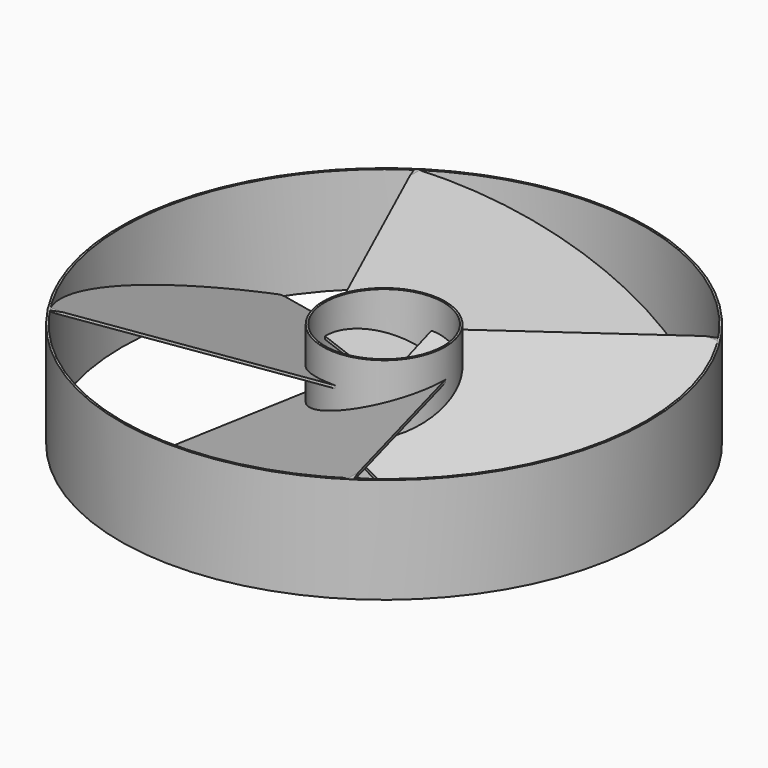
from build123d import *

# Parameters (mm, degrees)
F0_R      = 23.25
F0_R_2    = 22.5
F1_DEPTH  = 140
F3_R      = 100.25
F3_R_2    = 99.5
F4_DEPTH  = 40
F6_REACH  = 217.271158112
F8_DEPTH  = 50
F10_DEPTH = 150
F11_COUNT = 4
F14_ANGLE = 180
F15_R     = 43.2298787394
F16_DEPTH = 100


with BuildPart() as f1:
    # F0 (on Top) → F1 (new body)
    with BuildSketch(Plane.XY):
        Circle(F0_R)
        Circle(F0_R_2, mode=Mode.SUBTRACT)
    extrude(amount=F1_DEPTH)


with BuildPart() as f4:
    # F3 (on offset) → F4 (new body)
    with BuildSketch(Plane.XY.offset(140)):
        Circle(F3_R)
        Circle(F3_R_2, mode=Mode.SUBTRACT)
    extrude(amount=-F4_DEPTH)


with BuildPart() as f6:
    f6_end = f4.part.faces().sort_by_distance((-99.5, 0, 120))[0]
    # F5 (on Front) → F6 (new body, up to a face of F4 that its end follows)
    with BuildSketch(Plane.XZ):
        with BuildLine():
            Line((54.9857195201, 140), (53.5369125112, 140))
            Line((53.5369125112, 140), (-54.3417430631, 100.771397973))
            ThreePointArc((-54.3417430631, 100.771397973), (-54.7676606904, 100.4724610579), (-54.9857195201, 100))
            Line((-54.9857195201, 100), (-53.5369125112, 100))
            Line((-53.5369125112, 100), (54.3417430631, 139.228602027))
            ThreePointArc((54.3417430631, 139.228602027), (54.7676606904, 139.5275389421), (54.9857195201, 140))
        make_face()
    f6_long = extrude(amount=F6_REACH, mode=Mode.PRIVATE)
    add(split(f6_long, bisect_by=f6_end, keep=Keep.TOP, mode=Mode.PRIVATE))

    # F7 (on offset) → F8 (cut)
    with BuildSketch(Plane.XY.offset(140)):
        Polygon((-54.9857195201, -82.926597958), (-23.25, 0), (-54.3417430631, 0), (-54.9857195201, 0), align=None)
    extrude(amount=-F8_DEPTH, mode=Mode.SUBTRACT)

    # F9 (on Top) → F10 (cut)
    with BuildSketch(Plane.XY):
        Polygon((53.5369125112, 0), (23.25, 0), (54.9857195201, -82.926597958), (54.9857195201, -1e-10), align=None)
    extrude(amount=F10_DEPTH, mode=Mode.SUBTRACT)


with BuildPart() as f11_1:
    # F11: instance of F6
    add(f6.part.rotate(Axis((0, 0, 0), (0, 0, -1)), 1 * 360 / F11_COUNT))


with BuildPart() as f11_2:
    # F11: instance of F6
    add(f6.part.rotate(Axis((0, 0, 0), (0, 0, -1)), 2 * 360 / F11_COUNT))


with BuildPart() as f11_3:
    # F11: instance of F6
    add(f6.part.rotate(Axis((0, 0, 0), (0, 0, -1)), 3 * 360 / F11_COUNT))


with BuildPart() as f11_3_1:
    # F14: moved
    add(f11_3.part.rotate(Axis((26.6127046198, 0, 70), (1, 0, 0)), F14_ANGLE))


with BuildPart() as f1_1:
    # F14: moved
    add(f1.part.rotate(Axis((26.6127046198, 0, 70), (1, 0, 0)), F14_ANGLE))

    # F15 (on offset) → F16 (cut)
    with BuildSketch(Plane.XY.offset(140)):
        Circle(F15_R)
    extrude(amount=-F16_DEPTH, mode=Mode.SUBTRACT)


with BuildPart() as f6_1:
    # F14: moved
    add(f6.part.rotate(Axis((26.6127046198, 0, 70), (1, 0, 0)), F14_ANGLE))


with BuildPart() as f11_1_1:
    # F14: moved
    add(f11_1.part.rotate(Axis((26.6127046198, 0, 70), (1, 0, 0)), F14_ANGLE))


with BuildPart() as f4_1:
    # F14: moved
    add(f4.part.rotate(Axis((26.6127046198, 0, 70), (1, 0, 0)), F14_ANGLE))


with BuildPart() as f11_2_1:
    # F14: moved
    add(f11_2.part.rotate(Axis((26.6127046198, 0, 70), (1, 0, 0)), F14_ANGLE))


solid = Compound([f11_3_1.part, f1_1.part, f6_1.part, f11_1_1.part, f4_1.part, f11_2_1.part])
